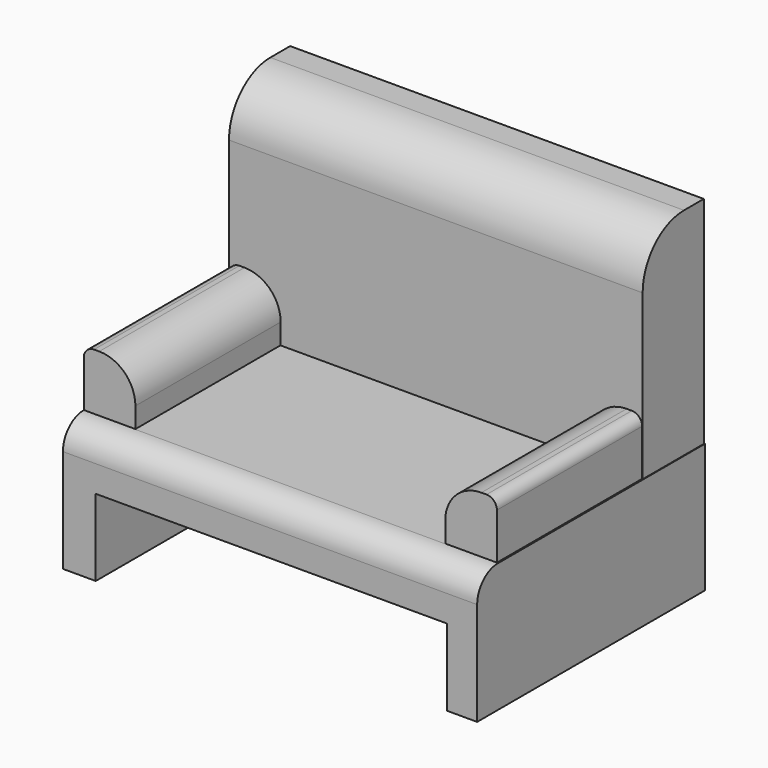
from build123d import *

# Parameters (mm, degrees)
F0_W      = 80.2132
F0_H      = 55.1688
F1_DEPTH  = 25
F3_W      = 80.0983905792
F3_H      = 66.7644366622
F4_DEPTH  = 14.8
F6_W      = 67.9705310613
F6_H      = 14.8716745898
F7_DEPTH  = 99
F8_R      = 5
F9_W      = 35.595134832
F9_H      = 10.9548680484
F10_DEPTH = 10
F11_R     = 7
F12_R     = 2
F13_R     = 10


# Not quite as in the source:
# - a pattern or mirror of a feature is missing from the dataset's text; its kind, count and spacing are read off the source's solid


with BuildPart() as f1:
    # F0 (on Top) → F1 (new body)
    with BuildSketch(Plane.XY):
        with Locations((40.1066, 27.5844)):
            Rectangle(F0_W, F0_H)
    extrude(amount=F1_DEPTH)

    # F3 (on offset) → F4 (join)
    with BuildSketch(Plane.XZ.offset(-55)):
        with Locations((40.0491952896, 33.3822183311)):
            Rectangle(F3_W, F3_H)
    extrude(amount=F4_DEPTH)

    # F6 (on Front) → F7 (cut)
    with BuildSketch(Plane.XZ):
        with Locations((40.3414806351, 7.4358372949)):
            Rectangle(F6_W, F6_H)
    extrude(amount=-F7_DEPTH, mode=Mode.SUBTRACT)

    # F8
    f8_edges = [f1.edges().sort_by_distance(p)[0] for p in [
        (40.1066, 0, 25),
    ]]
    fillet(f8_edges, radius=F8_R)

    # F9 (on Right) → F10 (join)
    with BuildSketch(Plane.YZ):
        with Locations((22.8417287581, 30.5123161525)):
            Rectangle(F9_W, F9_H)
    f10 = extrude(amount=F10_DEPTH)

    # F10_copies: F10 across plane
    add(f10.mirror(Plane(origin=(40, 0, 0), x_dir=(0, 0, 1), z_dir=(1, 0, 0))))

    # F11
    f11_edges = [f1.edges().sort_by_distance(p)[0] for p in [
        (10, 22.622081, 35.98975),
        (70, 22.622081, 35.98975),
    ]]
    fillet(f11_edges, radius=F11_R)

    # F12
    f12_edges = [f1.edges().sort_by_distance(p)[0] for p in [
        (0, 22.622081, 35.98975),
        (80, 22.622081, 35.98975),
    ]]
    fillet(f12_edges, radius=F12_R)

    # F13
    f13_edges = [f1.edges().sort_by_distance(p)[0] for p in [
        (40.049195, 40.2, 66.764437),
    ]]
    fillet(f13_edges, radius=F13_R)


solid = f1.part
